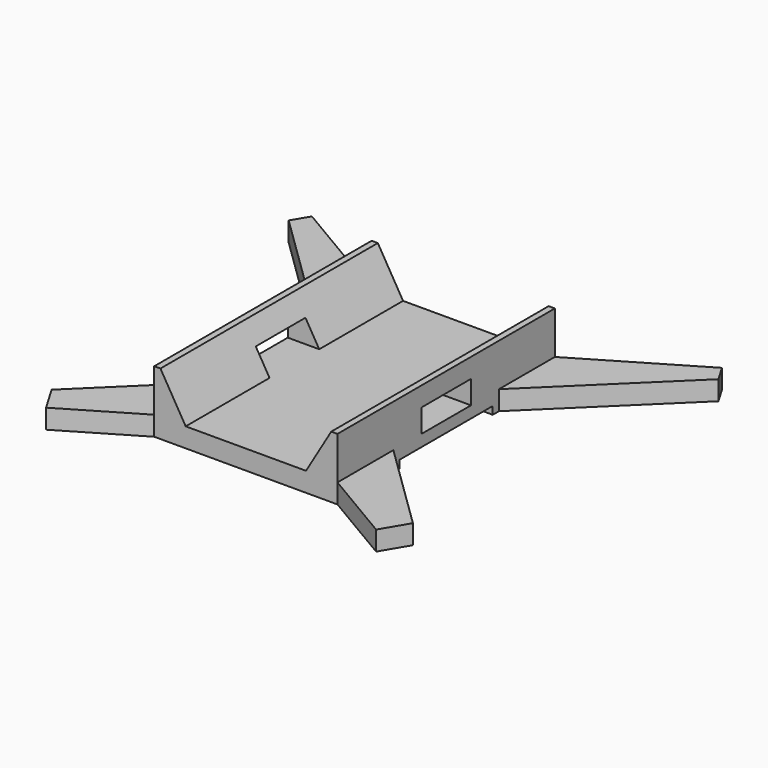
from build123d import *

# Parameters (mm, degrees)
F1_DEPTH = 17.5
F2_W     = 8
F2_H     = 3
F2_W_2   = 15
F2_H_2   = 1
F3_DEPTH = 50
F5_DEPTH = 2.5


# Not quite as in the source:
# - a pattern or mirror of a feature is missing from the dataset's text; its kind, count and spacing are read off the source's solid


with BuildPart() as f1:
    # F0 (on Front) → F1 (new body, symmetric)
    with BuildSketch(Plane.XZ):
        Polygon((-11.8, 0), (0, 0), (11.8, 0), (11.8, 8), (11, 8), (7.75, 2.5), (0, 2.5), (-7.75, 2.5), (-11, 8), (-11.8, 8), align=None)
    extrude(amount=F1_DEPTH, both=True)

    # F2 (on Right) → F3 (cut, symmetric)
    with BuildSketch(Plane.YZ):
        with Locations((0, 4)):
            Rectangle(F2_W, F2_H)
        with Locations((0, 0.5)):
            Rectangle(F2_W_2, F2_H_2)
    extrude(amount=F3_DEPTH, both=True, mode=Mode.SUBTRACT)

    # F4 (on Top) → F5 (join)
    with BuildSketch(Plane.XY):
        Polygon((26.4065545634, 26.1439538722), (11.8, 17.5), (11.8, 8.5), (27.6797758895, 23.9924642824), align=None)
        Polygon((11.8, -8.5), (11.8, -17.5), (21.2564246661, -23.0961793217), (23.2712739184, -19.6914867497), align=None)
    f5 = extrude(amount=F5_DEPTH)

    # F5_copies: F5 across plane
    add(f5.mirror(Plane(origin=(0, 0, 0), x_dir=(0, 0, -1), z_dir=(-1, 0, 0))))


solid = f1.part
